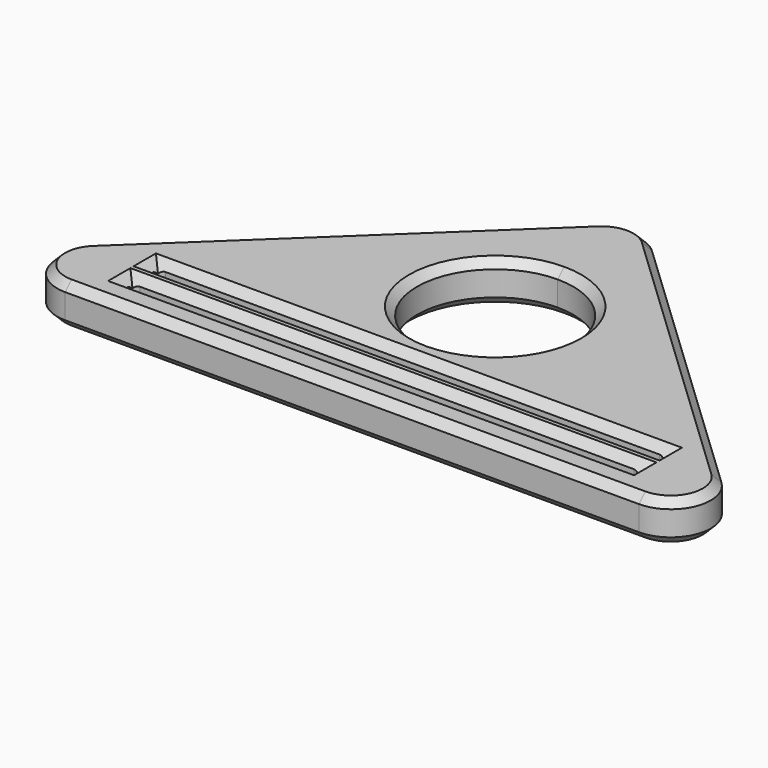
from build123d import *

# Parameters (mm, degrees)
F1_DEPTH      = 5.1
F2_R          = 5
F3_SIZE       = 1
F4_T4_DEPTH   = 8.1
F4_T10_DEPTH  = 8.1
F4_T16_DEPTH  = 8.1
F4_T24_DEPTH  = 8.1
F4_T30_DEPTH  = 8.1
F4_T36_DEPTH  = 8.1
F4_T42_DEPTH  = 8.1
F4_T48_DEPTH  = 8.1
F4_T56_DEPTH  = 8.1
F4_T62_DEPTH  = 8.1
F4_T68_DEPTH  = 8.1
F4_T74_DEPTH  = 8.1
F4_T80_DEPTH  = 8.1
F4_T88_DEPTH  = 8.1
F4_T94_DEPTH  = 8.1
F4_T100_DEPTH = 8.1
F4_T106_DEPTH = 8.1
F4_T112_DEPTH = 8.1
F4_T120_DEPTH = 8.1
F4_T126_DEPTH = 8.1
F4_T132_DEPTH = 8.1
F4_T138_DEPTH = 8.1
F4_T144_DEPTH = 8.1
F4_T152_DEPTH = 8.1
F4_T158_DEPTH = 8.1
F4_T164_DEPTH = 8.1
F4_T170_DEPTH = 8.1
F4_T176_DEPTH = 8.1
F4_T184_DEPTH = 8.1
F4_T190_DEPTH = 8.1
F4_T196_DEPTH = 8.1
F4_T202_DEPTH = 8.1
F4_T208_DEPTH = 8.1
F4_T216_DEPTH = 8.1
F4_T222_DEPTH = 8.1
F4_T228_DEPTH = 8.1
F4_T234_DEPTH = 8.1
F4_T240_DEPTH = 8.1
F4_T248_DEPTH = 8.1
F4_T254_DEPTH = 8.1


# Not quite as in the source:
# - a fillet or chamfer that OpenCascade refuses, or shapes differently, is made with other operations: its cross-section is extruded or revolved along the edge and cut away or added


with BuildPart() as f1:
    # F0 (on Top) → F1 (new body)
    with BuildSketch(Plane.XY):
        with BuildLine():
            Line((0, 2.5), (0, 0))
            Line((0, 0), (32, 0))
            Line((32, 0), (32, -1.5))
            Line((32, -1.5), (0, -1.5))
            Line((0, -1.5), (0, -5.4818979414))
            Line((0, -5.4818979414), (48.5503548798, -5.4818979414))
            Line((48.5503548798, -5.4818979414), (0, 40.5181020586))
            Line((0, 40.5181020586), (0, 26.7715353826))
            ThreePointArc((0, 26.7715353826), (6.9368136311, 23.8982130969), (9.8101359168, 16.9613994658))
            ThreePointArc((9.8101359168, 16.9613994658), (6.9368136311, 10.0245858347), (0, 7.151263549))
            Line((0, 7.151263549), (0, 4))
            Line((0, 4), (32, 4))
            Line((32, 4), (32, 2.5))
            Line((32, 2.5), (0, 2.5))
        make_face()
        with BuildLine():
            Line((-32, -1.5), (-32, 0))
            Line((-32, 0), (0, 0))
            Line((0, 0), (0, 2.5))
            Line((0, 2.5), (-32, 2.5))
            Line((-32, 2.5), (-32, 4))
            Line((-32, 4), (0, 4))
            Line((0, 4), (0, 7.151263549))
            ThreePointArc((0, 7.151263549), (-9.8101359168, 16.9613994658), (0, 26.7715353826))
            Line((0, 26.7715353826), (0, 40.5181020586))
            Line((0, 40.5181020586), (-48.5503548798, -5.4818979414))
            Line((-48.5503548798, -5.4818979414), (0, -5.4818979414))
            Line((0, -5.4818979414), (0, -1.5))
            Line((0, -1.5), (-32, -1.5))
        make_face()
    extrude(amount=F1_DEPTH)

    # F2
    f2_edges = [f1.edges().sort_by_distance(p)[0] for p in [
        (-48.550355, -5.481898, 2.55),
        (48.550355, -5.481898, 2.55),
        (0, 40.518102, 2.55),
    ]]
    fillet(f2_edges, radius=F2_R)

    # F3
    f3_edges = [f1.edges().sort_by_distance(p)[0] for p in [
        (21.440624, 20.203756, 5.1),
        (40.648189, -2.332857, 5.1),
        (0, 38.630252, 5.1),
        (0, -5.481898, 5.1),
        (-21.440624, 20.203756, 5.1),
        (-40.648189, -2.332857, 5.1),
        (32, 3.25, 5.1),
        (0, 2.5, 5.1),
        (-32, 3.25, 5.1),
        (0, 4, 5.1),
        (32, -0.75, 5.1),
        (0, -1.5, 5.1),
        (-32, -0.75, 5.1),
        (0, 0, 5.1),
        (-9.810136, 16.961399, 5.1),
        (21.440624, 20.203756, 0),
        (40.648189, -2.332857, 0),
        (0, 38.630252, 0),
        (0, -5.481898, 0),
        (-21.440624, 20.203756, 0),
        (-40.648189, -2.332857, 0),
        (32, 3.25, 0),
        (0, 2.5, 0),
        (-32, 3.25, 0),
        (0, 4, 0),
        (32, -0.75, 0),
        (0, -1.5, 0),
        (-32, -0.75, 0),
        (0, 0, 0),
        (-9.810136, 16.961399, 0),
    ]]
    chamfer(f3_edges, length=F3_SIZE)

    # F4: fillet of radius 1 on 8 edges, made by hand


with BuildPart() as f4_tool2:
    # F4_s3 → F4_t4 (new body)
    with BuildSketch(Plane.XY.offset(-1.5)):
        with BuildLine():
            ThreePointArc((32, 3.5), (31.7071067812, 2.7928932188), (31, 2.5))
            Line((31, 2.5), (32, 2.5))
            Line((32, 2.5), (32, 3.5))
        make_face()
    extrude(amount=F4_T4_DEPTH)

    split(bisect_by=Plane(origin=(16.5, 0, 16.5), x_dir=(0, 1, 0), z_dir=(-0.7071067812, 0, -0.7071067812)), keep=Keep.TOP)

    split(bisect_by=Plane(origin=(0, 0.75, -0.75), x_dir=(1, 0, 0), z_dir=(0, -0.7071067812, 0.7071067812)), keep=Keep.TOP)


with BuildPart() as f1_1:
    add(f1.part)

    # F4_t1: union F4_tool2
    add(f4_tool2.part)


with BuildPart() as f4_tool8:
    # F4_s9 → F4_t10 (new body)
    with BuildSketch(Plane.XY.offset(-1.5)):
        with BuildLine():
            ThreePointArc((32, 3.5), (31.7071067812, 2.7928932188), (31, 2.5))
            Line((31, 2.5), (32, 2.5))
            Line((32, 2.5), (32, 3.5))
        make_face()
    extrude(amount=F4_T10_DEPTH)

    split(bisect_by=Plane(origin=(16.5, 0, 16.5), x_dir=(0, 1, 0), z_dir=(0.7071067812, 0, 0.7071067812)), keep=Keep.TOP)

    split(bisect_by=Plane(origin=(0, 0.75, -0.75), x_dir=(1, 0, 0), z_dir=(0, 0.7071067812, -0.7071067812)), keep=Keep.TOP)


with BuildPart() as f1_2:
    add(f1_1.part)

    # F4_t7: union F4_tool8
    add(f4_tool8.part)


with BuildPart() as f4_tool14:
    # F4_s15 → F4_t16 (new body)
    with BuildSketch(Plane.XY.offset(-1.5)):
        with BuildLine():
            ThreePointArc((32, 3.5), (31.7071067812, 2.7928932188), (31, 2.5))
            Line((31, 2.5), (32, 2.5))
            Line((32, 2.5), (32, 3.5))
        make_face()
    extrude(amount=F4_T16_DEPTH)

    split(bisect_by=Plane(origin=(16.5, 0, 16.5), x_dir=(0, 1, 0), z_dir=(0.7071067812, 0, 0.7071067812)), keep=Keep.TOP)

    split(bisect_by=Plane(origin=(0, 0.75, -0.75), x_dir=(1, 0, 0), z_dir=(0, -0.7071067812, 0.7071067812)), keep=Keep.TOP)

    split(bisect_by=Plane(origin=(13.95, 0, -13.95), x_dir=(0, 1, 0), z_dir=(0.7071067812, 0, -0.7071067812)), keep=Keep.TOP)

    split(bisect_by=Plane(origin=(0, 3.3, 3.3), x_dir=(1, 0, 0), z_dir=(0, -0.7071067812, -0.7071067812)), keep=Keep.TOP)


with BuildPart() as f1_3:
    add(f1_2.part)

    # F4_t13: union F4_tool14
    add(f4_tool14.part)


with BuildPart() as f4_tool22:
    # F4_s23 → F4_t24 (new body)
    with BuildSketch(Plane.XY.offset(-1.5)):
        with BuildLine():
            ThreePointArc((32, 3.5), (31.7071067812, 2.7928932188), (31, 2.5))
            Line((31, 2.5), (32, 2.5))
            Line((32, 2.5), (32, 3.5))
        make_face()
    extrude(amount=F4_T24_DEPTH)

    split(bisect_by=Plane(origin=(13.95, 0, -13.95), x_dir=(0, 1, 0), z_dir=(-0.7071067812, 0, 0.7071067812)), keep=Keep.TOP)

    split(bisect_by=Plane(origin=(0, 3.3, 3.3), x_dir=(1, 0, 0), z_dir=(0, -0.7071067812, -0.7071067812)), keep=Keep.TOP)


with BuildPart() as f1_4:
    add(f1_3.part)

    # F4_t21: union F4_tool22
    add(f4_tool22.part)


with BuildPart() as f4_tool28:
    # F4_s29 → F4_t30 (new body)
    with BuildSketch(Plane.XY.offset(-1.5)):
        with BuildLine():
            ThreePointArc((32, 3.5), (31.7071067812, 2.7928932188), (31, 2.5))
            Line((31, 2.5), (32, 2.5))
            Line((32, 2.5), (32, 3.5))
        make_face()
    extrude(amount=F4_T30_DEPTH)

    split(bisect_by=Plane(origin=(13.95, 0, -13.95), x_dir=(0, 1, 0), z_dir=(0.7071067812, 0, -0.7071067812)), keep=Keep.TOP)

    split(bisect_by=Plane(origin=(0, 3.3, 3.3), x_dir=(1, 0, 0), z_dir=(0, 0.7071067812, 0.7071067812)), keep=Keep.TOP)


with BuildPart() as f1_5:
    add(f1_4.part)

    # F4_t27: union F4_tool28
    add(f4_tool28.part)


with BuildPart() as f4_tool34:
    # F4_s35 → F4_t36 (new body)
    with BuildSketch(Plane.XY.offset(-1.5)):
        with BuildLine():
            ThreePointArc((32, -1), (31.7071067812, -0.2928932188), (31, 0))
            Line((31, 0), (32, 0))
            Line((32, 0), (32, -1))
        make_face()
    extrude(amount=F4_T36_DEPTH)

    split(bisect_by=Plane(origin=(16.5, 0, 16.5), x_dir=(0, 1, 0), z_dir=(-0.7071067812, 0, -0.7071067812)), keep=Keep.TOP)

    split(bisect_by=Plane(origin=(0, 0.5, 0.5), x_dir=(1, 0, 0), z_dir=(0, 0.7071067812, 0.7071067812)), keep=Keep.TOP)


with BuildPart() as f1_6:
    add(f1_5.part)

    # F4_t33: union F4_tool34
    add(f4_tool34.part)


with BuildPart() as f4_tool40:
    # F4_s41 → F4_t42 (new body)
    with BuildSketch(Plane.XY.offset(-1.5)):
        with BuildLine():
            ThreePointArc((32, -1), (31.7071067812, -0.2928932188), (31, 0))
            Line((31, 0), (32, 0))
            Line((32, 0), (32, -1))
        make_face()
    extrude(amount=F4_T42_DEPTH)

    split(bisect_by=Plane(origin=(16.5, 0, 16.5), x_dir=(0, 1, 0), z_dir=(0.7071067812, 0, 0.7071067812)), keep=Keep.TOP)

    split(bisect_by=Plane(origin=(0, 0.5, 0.5), x_dir=(1, 0, 0), z_dir=(0, -0.7071067812, -0.7071067812)), keep=Keep.TOP)


with BuildPart() as f1_7:
    add(f1_6.part)

    # F4_t39: union F4_tool40
    add(f4_tool40.part)


with BuildPart() as f4_tool46:
    # F4_s47 → F4_t48 (new body)
    with BuildSketch(Plane.XY.offset(-1.5)):
        with BuildLine():
            ThreePointArc((32, -1), (31.7071067812, -0.2928932188), (31, 0))
            Line((31, 0), (32, 0))
            Line((32, 0), (32, -1))
        make_face()
    extrude(amount=F4_T48_DEPTH)

    split(bisect_by=Plane(origin=(16.5, 0, 16.5), x_dir=(0, 1, 0), z_dir=(0.7071067812, 0, 0.7071067812)), keep=Keep.TOP)

    split(bisect_by=Plane(origin=(0, 0.5, 0.5), x_dir=(1, 0, 0), z_dir=(0, 0.7071067812, 0.7071067812)), keep=Keep.TOP)

    split(bisect_by=Plane(origin=(13.95, 0, -13.95), x_dir=(0, 1, 0), z_dir=(0.7071067812, 0, -0.7071067812)), keep=Keep.TOP)

    split(bisect_by=Plane(origin=(0, -2.05, 2.05), x_dir=(1, 0, 0), z_dir=(0, 0.7071067812, -0.7071067812)), keep=Keep.TOP)


with BuildPart() as f1_8:
    add(f1_7.part)

    # F4_t45: union F4_tool46
    add(f4_tool46.part)


with BuildPart() as f4_tool54:
    # F4_s55 → F4_t56 (new body)
    with BuildSketch(Plane.XY.offset(-1.5)):
        with BuildLine():
            ThreePointArc((32, -1), (31.7071067812, -0.2928932188), (31, 0))
            Line((31, 0), (32, 0))
            Line((32, 0), (32, -1))
        make_face()
    extrude(amount=F4_T56_DEPTH)

    split(bisect_by=Plane(origin=(13.95, 0, -13.95), x_dir=(0, 1, 0), z_dir=(-0.7071067812, 0, 0.7071067812)), keep=Keep.TOP)

    split(bisect_by=Plane(origin=(0, -2.05, 2.05), x_dir=(1, 0, 0), z_dir=(0, 0.7071067812, -0.7071067812)), keep=Keep.TOP)


with BuildPart() as f1_9:
    add(f1_8.part)

    # F4_t53: union F4_tool54
    add(f4_tool54.part)


with BuildPart() as f4_tool60:
    # F4_s61 → F4_t62 (new body)
    with BuildSketch(Plane.XY.offset(-1.5)):
        with BuildLine():
            ThreePointArc((32, -1), (31.7071067812, -0.2928932188), (31, 0))
            Line((31, 0), (32, 0))
            Line((32, 0), (32, -1))
        make_face()
    extrude(amount=F4_T62_DEPTH)

    split(bisect_by=Plane(origin=(13.95, 0, -13.95), x_dir=(0, 1, 0), z_dir=(0.7071067812, 0, -0.7071067812)), keep=Keep.TOP)

    split(bisect_by=Plane(origin=(0, -2.05, 2.05), x_dir=(1, 0, 0), z_dir=(0, -0.7071067812, 0.7071067812)), keep=Keep.TOP)


with BuildPart() as f1_10:
    add(f1_9.part)

    # F4_t59: union F4_tool60
    add(f4_tool60.part)


with BuildPart() as f4_tool66:
    # F4_s67 → F4_t68 (new body)
    with BuildSketch(Plane.XY.offset(-1.5)):
        with BuildLine():
            ThreePointArc((32, -0.5), (31.7071067812, -1.2071067812), (31, -1.5))
            Line((31, -1.5), (32, -1.5))
            Line((32, -1.5), (32, -0.5))
        make_face()
    extrude(amount=F4_T68_DEPTH)

    split(bisect_by=Plane(origin=(16.5, 0, 16.5), x_dir=(0, 1, 0), z_dir=(-0.7071067812, 0, -0.7071067812)), keep=Keep.TOP)

    split(bisect_by=Plane(origin=(0, -1.25, 1.25), x_dir=(1, 0, 0), z_dir=(0, -0.7071067812, 0.7071067812)), keep=Keep.TOP)


with BuildPart() as f1_11:
    add(f1_10.part)

    # F4_t65: union F4_tool66
    add(f4_tool66.part)


with BuildPart() as f4_tool72:
    # F4_s73 → F4_t74 (new body)
    with BuildSketch(Plane.XY.offset(-1.5)):
        with BuildLine():
            ThreePointArc((32, -0.5), (31.7071067812, -1.2071067812), (31, -1.5))
            Line((31, -1.5), (32, -1.5))
            Line((32, -1.5), (32, -0.5))
        make_face()
    extrude(amount=F4_T74_DEPTH)

    split(bisect_by=Plane(origin=(16.5, 0, 16.5), x_dir=(0, 1, 0), z_dir=(0.7071067812, 0, 0.7071067812)), keep=Keep.TOP)

    split(bisect_by=Plane(origin=(0, -1.25, 1.25), x_dir=(1, 0, 0), z_dir=(0, 0.7071067812, -0.7071067812)), keep=Keep.TOP)


with BuildPart() as f1_12:
    add(f1_11.part)

    # F4_t71: union F4_tool72
    add(f4_tool72.part)


with BuildPart() as f4_tool78:
    # F4_s79 → F4_t80 (new body)
    with BuildSketch(Plane.XY.offset(-1.5)):
        with BuildLine():
            ThreePointArc((32, -0.5), (31.7071067812, -1.2071067812), (31, -1.5))
            Line((31, -1.5), (32, -1.5))
            Line((32, -1.5), (32, -0.5))
        make_face()
    extrude(amount=F4_T80_DEPTH)

    split(bisect_by=Plane(origin=(16.5, 0, 16.5), x_dir=(0, 1, 0), z_dir=(0.7071067812, 0, 0.7071067812)), keep=Keep.TOP)

    split(bisect_by=Plane(origin=(0, -1.25, 1.25), x_dir=(1, 0, 0), z_dir=(0, -0.7071067812, 0.7071067812)), keep=Keep.TOP)

    split(bisect_by=Plane(origin=(13.95, 0, -13.95), x_dir=(0, 1, 0), z_dir=(0.7071067812, 0, -0.7071067812)), keep=Keep.TOP)

    split(bisect_by=Plane(origin=(0, 1.3, 1.3), x_dir=(1, 0, 0), z_dir=(0, -0.7071067812, -0.7071067812)), keep=Keep.TOP)


with BuildPart() as f1_13:
    add(f1_12.part)

    # F4_t77: union F4_tool78
    add(f4_tool78.part)


with BuildPart() as f4_tool86:
    # F4_s87 → F4_t88 (new body)
    with BuildSketch(Plane.XY.offset(-1.5)):
        with BuildLine():
            ThreePointArc((32, -0.5), (31.7071067812, -1.2071067812), (31, -1.5))
            Line((31, -1.5), (32, -1.5))
            Line((32, -1.5), (32, -0.5))
        make_face()
    extrude(amount=F4_T88_DEPTH)

    split(bisect_by=Plane(origin=(13.95, 0, -13.95), x_dir=(0, 1, 0), z_dir=(-0.7071067812, 0, 0.7071067812)), keep=Keep.TOP)

    split(bisect_by=Plane(origin=(0, 1.3, 1.3), x_dir=(1, 0, 0), z_dir=(0, -0.7071067812, -0.7071067812)), keep=Keep.TOP)


with BuildPart() as f1_14:
    add(f1_13.part)

    # F4_t85: union F4_tool86
    add(f4_tool86.part)


with BuildPart() as f4_tool92:
    # F4_s93 → F4_t94 (new body)
    with BuildSketch(Plane.XY.offset(-1.5)):
        with BuildLine():
            ThreePointArc((32, -0.5), (31.7071067812, -1.2071067812), (31, -1.5))
            Line((31, -1.5), (32, -1.5))
            Line((32, -1.5), (32, -0.5))
        make_face()
    extrude(amount=F4_T94_DEPTH)

    split(bisect_by=Plane(origin=(13.95, 0, -13.95), x_dir=(0, 1, 0), z_dir=(0.7071067812, 0, -0.7071067812)), keep=Keep.TOP)

    split(bisect_by=Plane(origin=(0, 1.3, 1.3), x_dir=(1, 0, 0), z_dir=(0, 0.7071067812, 0.7071067812)), keep=Keep.TOP)


with BuildPart() as f1_15:
    add(f1_14.part)

    # F4_t91: union F4_tool92
    add(f4_tool92.part)


with BuildPart() as f4_tool98:
    # F4_s99 → F4_t100 (new body)
    with BuildSketch(Plane.XY.offset(-1.5)):
        with BuildLine():
            ThreePointArc((32, 3), (31.7071067812, 3.7071067812), (31, 4))
            Line((31, 4), (32, 4))
            Line((32, 4), (32, 3))
        make_face()
    extrude(amount=F4_T100_DEPTH)

    split(bisect_by=Plane(origin=(16.5, 0, 16.5), x_dir=(0, 1, 0), z_dir=(-0.7071067812, 0, -0.7071067812)), keep=Keep.TOP)

    split(bisect_by=Plane(origin=(0, 2.5, 2.5), x_dir=(1, 0, 0), z_dir=(0, 0.7071067812, 0.7071067812)), keep=Keep.TOP)


with BuildPart() as f1_16:
    add(f1_15.part)

    # F4_t97: union F4_tool98
    add(f4_tool98.part)


with BuildPart() as f4_tool104:
    # F4_s105 → F4_t106 (new body)
    with BuildSketch(Plane.XY.offset(-1.5)):
        with BuildLine():
            ThreePointArc((32, 3), (31.7071067812, 3.7071067812), (31, 4))
            Line((31, 4), (32, 4))
            Line((32, 4), (32, 3))
        make_face()
    extrude(amount=F4_T106_DEPTH)

    split(bisect_by=Plane(origin=(16.5, 0, 16.5), x_dir=(0, 1, 0), z_dir=(0.7071067812, 0, 0.7071067812)), keep=Keep.TOP)

    split(bisect_by=Plane(origin=(0, 2.5, 2.5), x_dir=(1, 0, 0), z_dir=(0, -0.7071067812, -0.7071067812)), keep=Keep.TOP)


with BuildPart() as f1_17:
    add(f1_16.part)

    # F4_t103: union F4_tool104
    add(f4_tool104.part)


with BuildPart() as f4_tool110:
    # F4_s111 → F4_t112 (new body)
    with BuildSketch(Plane.XY.offset(-1.5)):
        with BuildLine():
            ThreePointArc((32, 3), (31.7071067812, 3.7071067812), (31, 4))
            Line((31, 4), (32, 4))
            Line((32, 4), (32, 3))
        make_face()
    extrude(amount=F4_T112_DEPTH)

    split(bisect_by=Plane(origin=(16.5, 0, 16.5), x_dir=(0, 1, 0), z_dir=(0.7071067812, 0, 0.7071067812)), keep=Keep.TOP)

    split(bisect_by=Plane(origin=(0, 2.5, 2.5), x_dir=(1, 0, 0), z_dir=(0, 0.7071067812, 0.7071067812)), keep=Keep.TOP)

    split(bisect_by=Plane(origin=(13.95, 0, -13.95), x_dir=(0, 1, 0), z_dir=(0.7071067812, 0, -0.7071067812)), keep=Keep.TOP)

    split(bisect_by=Plane(origin=(0, -0.05, 0.05), x_dir=(1, 0, 0), z_dir=(0, 0.7071067812, -0.7071067812)), keep=Keep.TOP)


with BuildPart() as f1_18:
    add(f1_17.part)

    # F4_t109: union F4_tool110
    add(f4_tool110.part)


with BuildPart() as f4_tool118:
    # F4_s119 → F4_t120 (new body)
    with BuildSketch(Plane.XY.offset(-1.5)):
        with BuildLine():
            ThreePointArc((32, 3), (31.7071067812, 3.7071067812), (31, 4))
            Line((31, 4), (32, 4))
            Line((32, 4), (32, 3))
        make_face()
    extrude(amount=F4_T120_DEPTH)

    split(bisect_by=Plane(origin=(13.95, 0, -13.95), x_dir=(0, 1, 0), z_dir=(-0.7071067812, 0, 0.7071067812)), keep=Keep.TOP)

    split(bisect_by=Plane(origin=(0, -0.05, 0.05), x_dir=(1, 0, 0), z_dir=(0, 0.7071067812, -0.7071067812)), keep=Keep.TOP)


with BuildPart() as f1_19:
    add(f1_18.part)

    # F4_t117: union F4_tool118
    add(f4_tool118.part)


with BuildPart() as f4_tool124:
    # F4_s125 → F4_t126 (new body)
    with BuildSketch(Plane.XY.offset(-1.5)):
        with BuildLine():
            ThreePointArc((32, 3), (31.7071067812, 3.7071067812), (31, 4))
            Line((31, 4), (32, 4))
            Line((32, 4), (32, 3))
        make_face()
    extrude(amount=F4_T126_DEPTH)

    split(bisect_by=Plane(origin=(13.95, 0, -13.95), x_dir=(0, 1, 0), z_dir=(0.7071067812, 0, -0.7071067812)), keep=Keep.TOP)

    split(bisect_by=Plane(origin=(0, -0.05, 0.05), x_dir=(1, 0, 0), z_dir=(0, -0.7071067812, 0.7071067812)), keep=Keep.TOP)


with BuildPart() as f1_20:
    add(f1_19.part)

    # F4_t123: union F4_tool124
    add(f4_tool124.part)


with BuildPart() as f4_tool130:
    # F4_s131 → F4_t132 (new body)
    with BuildSketch(Plane.XY.offset(-1.5)):
        with BuildLine():
            ThreePointArc((-31, -1.5), (-31.7071067812, -1.2071067812), (-32, -0.5))
            Line((-32, -0.5), (-32, -1.5))
            Line((-32, -1.5), (-31, -1.5))
        make_face()
    extrude(amount=F4_T132_DEPTH)

    split(bisect_by=Plane(origin=(0, -1.25, 1.25), x_dir=(1, 0, 0), z_dir=(0, 0.7071067812, -0.7071067812)), keep=Keep.TOP)

    split(bisect_by=Plane(origin=(-16.5, 0, 16.5), x_dir=(0, 1, 0), z_dir=(-0.7071067812, 0, 0.7071067812)), keep=Keep.TOP)


with BuildPart() as f1_21:
    add(f1_20.part)

    # F4_t129: union F4_tool130
    add(f4_tool130.part)


with BuildPart() as f4_tool136:
    # F4_s137 → F4_t138 (new body)
    with BuildSketch(Plane.XY.offset(-1.5)):
        with BuildLine():
            ThreePointArc((-31, -1.5), (-31.7071067812, -1.2071067812), (-32, -0.5))
            Line((-32, -0.5), (-32, -1.5))
            Line((-32, -1.5), (-31, -1.5))
        make_face()
    extrude(amount=F4_T138_DEPTH)

    split(bisect_by=Plane(origin=(0, -1.25, 1.25), x_dir=(1, 0, 0), z_dir=(0, -0.7071067812, 0.7071067812)), keep=Keep.TOP)

    split(bisect_by=Plane(origin=(-16.5, 0, 16.5), x_dir=(0, 1, 0), z_dir=(0.7071067812, 0, -0.7071067812)), keep=Keep.TOP)


with BuildPart() as f1_22:
    add(f1_21.part)

    # F4_t135: union F4_tool136
    add(f4_tool136.part)


with BuildPart() as f4_tool142:
    # F4_s143 → F4_t144 (new body)
    with BuildSketch(Plane.XY.offset(-1.5)):
        with BuildLine():
            ThreePointArc((-31, -1.5), (-31.7071067812, -1.2071067812), (-32, -0.5))
            Line((-32, -0.5), (-32, -1.5))
            Line((-32, -1.5), (-31, -1.5))
        make_face()
    extrude(amount=F4_T144_DEPTH)

    split(bisect_by=Plane(origin=(0, -1.25, 1.25), x_dir=(1, 0, 0), z_dir=(0, -0.7071067812, 0.7071067812)), keep=Keep.TOP)

    split(bisect_by=Plane(origin=(-16.5, 0, 16.5), x_dir=(0, 1, 0), z_dir=(-0.7071067812, 0, 0.7071067812)), keep=Keep.TOP)

    split(bisect_by=Plane(origin=(0, 1.3, 1.3), x_dir=(1, 0, 0), z_dir=(0, -0.7071067812, -0.7071067812)), keep=Keep.TOP)

    split(bisect_by=Plane(origin=(-13.95, 0, -13.95), x_dir=(0, 1, 0), z_dir=(-0.7071067812, 0, -0.7071067812)), keep=Keep.TOP)


with BuildPart() as f1_23:
    add(f1_22.part)

    # F4_t141: union F4_tool142
    add(f4_tool142.part)


with BuildPart() as f4_tool150:
    # F4_s151 → F4_t152 (new body)
    with BuildSketch(Plane.XY.offset(-1.5)):
        with BuildLine():
            ThreePointArc((-31, -1.5), (-31.7071067812, -1.2071067812), (-32, -0.5))
            Line((-32, -0.5), (-32, -1.5))
            Line((-32, -1.5), (-31, -1.5))
        make_face()
    extrude(amount=F4_T152_DEPTH)

    split(bisect_by=Plane(origin=(0, 1.3, 1.3), x_dir=(1, 0, 0), z_dir=(0, 0.7071067812, 0.7071067812)), keep=Keep.TOP)

    split(bisect_by=Plane(origin=(-13.95, 0, -13.95), x_dir=(0, 1, 0), z_dir=(-0.7071067812, 0, -0.7071067812)), keep=Keep.TOP)


with BuildPart() as f1_24:
    add(f1_23.part)

    # F4_t149: union F4_tool150
    add(f4_tool150.part)


with BuildPart() as f4_tool156:
    # F4_s157 → F4_t158 (new body)
    with BuildSketch(Plane.XY.offset(-1.5)):
        with BuildLine():
            ThreePointArc((-31, -1.5), (-31.7071067812, -1.2071067812), (-32, -0.5))
            Line((-32, -0.5), (-32, -1.5))
            Line((-32, -1.5), (-31, -1.5))
        make_face()
    extrude(amount=F4_T158_DEPTH)

    split(bisect_by=Plane(origin=(0, 1.3, 1.3), x_dir=(1, 0, 0), z_dir=(0, -0.7071067812, -0.7071067812)), keep=Keep.TOP)

    split(bisect_by=Plane(origin=(-13.95, 0, -13.95), x_dir=(0, 1, 0), z_dir=(0.7071067812, 0, 0.7071067812)), keep=Keep.TOP)


with BuildPart() as f1_25:
    add(f1_24.part)

    # F4_t155: union F4_tool156
    add(f4_tool156.part)


with BuildPart() as f4_tool162:
    # F4_s163 → F4_t164 (new body)
    with BuildSketch(Plane.XY.offset(-1.5)):
        with BuildLine():
            ThreePointArc((-31, 2.5), (-31.7071067812, 2.7928932188), (-32, 3.5))
            Line((-32, 3.5), (-32, 2.5))
            Line((-32, 2.5), (-31, 2.5))
        make_face()
    extrude(amount=F4_T164_DEPTH)

    split(bisect_by=Plane(origin=(0, 0.75, -0.75), x_dir=(1, 0, 0), z_dir=(0, 0.7071067812, -0.7071067812)), keep=Keep.TOP)

    split(bisect_by=Plane(origin=(-16.5, 0, 16.5), x_dir=(0, 1, 0), z_dir=(-0.7071067812, 0, 0.7071067812)), keep=Keep.TOP)


with BuildPart() as f1_26:
    add(f1_25.part)

    # F4_t161: union F4_tool162
    add(f4_tool162.part)


with BuildPart() as f4_tool168:
    # F4_s169 → F4_t170 (new body)
    with BuildSketch(Plane.XY.offset(-1.5)):
        with BuildLine():
            ThreePointArc((-31, 2.5), (-31.7071067812, 2.7928932188), (-32, 3.5))
            Line((-32, 3.5), (-32, 2.5))
            Line((-32, 2.5), (-31, 2.5))
        make_face()
    extrude(amount=F4_T170_DEPTH)

    split(bisect_by=Plane(origin=(0, 0.75, -0.75), x_dir=(1, 0, 0), z_dir=(0, -0.7071067812, 0.7071067812)), keep=Keep.TOP)

    split(bisect_by=Plane(origin=(-16.5, 0, 16.5), x_dir=(0, 1, 0), z_dir=(0.7071067812, 0, -0.7071067812)), keep=Keep.TOP)


with BuildPart() as f1_27:
    add(f1_26.part)

    # F4_t167: union F4_tool168
    add(f4_tool168.part)


with BuildPart() as f4_tool174:
    # F4_s175 → F4_t176 (new body)
    with BuildSketch(Plane.XY.offset(-1.5)):
        with BuildLine():
            ThreePointArc((-31, 2.5), (-31.7071067812, 2.7928932188), (-32, 3.5))
            Line((-32, 3.5), (-32, 2.5))
            Line((-32, 2.5), (-31, 2.5))
        make_face()
    extrude(amount=F4_T176_DEPTH)

    split(bisect_by=Plane(origin=(0, 0.75, -0.75), x_dir=(1, 0, 0), z_dir=(0, -0.7071067812, 0.7071067812)), keep=Keep.TOP)

    split(bisect_by=Plane(origin=(-16.5, 0, 16.5), x_dir=(0, 1, 0), z_dir=(-0.7071067812, 0, 0.7071067812)), keep=Keep.TOP)

    split(bisect_by=Plane(origin=(0, 3.3, 3.3), x_dir=(1, 0, 0), z_dir=(0, -0.7071067812, -0.7071067812)), keep=Keep.TOP)

    split(bisect_by=Plane(origin=(-13.95, 0, -13.95), x_dir=(0, 1, 0), z_dir=(-0.7071067812, 0, -0.7071067812)), keep=Keep.TOP)


with BuildPart() as f1_28:
    add(f1_27.part)

    # F4_t173: union F4_tool174
    add(f4_tool174.part)


with BuildPart() as f4_tool182:
    # F4_s183 → F4_t184 (new body)
    with BuildSketch(Plane.XY.offset(-1.5)):
        with BuildLine():
            ThreePointArc((-31, 2.5), (-31.7071067812, 2.7928932188), (-32, 3.5))
            Line((-32, 3.5), (-32, 2.5))
            Line((-32, 2.5), (-31, 2.5))
        make_face()
    extrude(amount=F4_T184_DEPTH)

    split(bisect_by=Plane(origin=(0, 3.3, 3.3), x_dir=(1, 0, 0), z_dir=(0, 0.7071067812, 0.7071067812)), keep=Keep.TOP)

    split(bisect_by=Plane(origin=(-13.95, 0, -13.95), x_dir=(0, 1, 0), z_dir=(-0.7071067812, 0, -0.7071067812)), keep=Keep.TOP)


with BuildPart() as f1_29:
    add(f1_28.part)

    # F4_t181: union F4_tool182
    add(f4_tool182.part)


with BuildPart() as f4_tool188:
    # F4_s189 → F4_t190 (new body)
    with BuildSketch(Plane.XY.offset(-1.5)):
        with BuildLine():
            ThreePointArc((-31, 2.5), (-31.7071067812, 2.7928932188), (-32, 3.5))
            Line((-32, 3.5), (-32, 2.5))
            Line((-32, 2.5), (-31, 2.5))
        make_face()
    extrude(amount=F4_T190_DEPTH)

    split(bisect_by=Plane(origin=(0, 3.3, 3.3), x_dir=(1, 0, 0), z_dir=(0, -0.7071067812, -0.7071067812)), keep=Keep.TOP)

    split(bisect_by=Plane(origin=(-13.95, 0, -13.95), x_dir=(0, 1, 0), z_dir=(0.7071067812, 0, 0.7071067812)), keep=Keep.TOP)


with BuildPart() as f1_30:
    add(f1_29.part)

    # F4_t187: union F4_tool188
    add(f4_tool188.part)


with BuildPart() as f4_tool194:
    # F4_s195 → F4_t196 (new body)
    with BuildSketch(Plane.XY.offset(-1.5)):
        with BuildLine():
            ThreePointArc((-31, 4), (-31.7071067812, 3.7071067812), (-32, 3))
            Line((-32, 3), (-32, 4))
            Line((-32, 4), (-31, 4))
        make_face()
    extrude(amount=F4_T196_DEPTH)

    split(bisect_by=Plane(origin=(0, 2.5, 2.5), x_dir=(1, 0, 0), z_dir=(0, -0.7071067812, -0.7071067812)), keep=Keep.TOP)

    split(bisect_by=Plane(origin=(-16.5, 0, 16.5), x_dir=(0, 1, 0), z_dir=(-0.7071067812, 0, 0.7071067812)), keep=Keep.TOP)


with BuildPart() as f1_31:
    add(f1_30.part)

    # F4_t193: union F4_tool194
    add(f4_tool194.part)


with BuildPart() as f4_tool200:
    # F4_s201 → F4_t202 (new body)
    with BuildSketch(Plane.XY.offset(-1.5)):
        with BuildLine():
            ThreePointArc((-31, 4), (-31.7071067812, 3.7071067812), (-32, 3))
            Line((-32, 3), (-32, 4))
            Line((-32, 4), (-31, 4))
        make_face()
    extrude(amount=F4_T202_DEPTH)

    split(bisect_by=Plane(origin=(0, 2.5, 2.5), x_dir=(1, 0, 0), z_dir=(0, 0.7071067812, 0.7071067812)), keep=Keep.TOP)

    split(bisect_by=Plane(origin=(-16.5, 0, 16.5), x_dir=(0, 1, 0), z_dir=(0.7071067812, 0, -0.7071067812)), keep=Keep.TOP)


with BuildPart() as f1_32:
    add(f1_31.part)

    # F4_t199: union F4_tool200
    add(f4_tool200.part)


with BuildPart() as f4_tool206:
    # F4_s207 → F4_t208 (new body)
    with BuildSketch(Plane.XY.offset(-1.5)):
        with BuildLine():
            ThreePointArc((-31, 4), (-31.7071067812, 3.7071067812), (-32, 3))
            Line((-32, 3), (-32, 4))
            Line((-32, 4), (-31, 4))
        make_face()
    extrude(amount=F4_T208_DEPTH)

    split(bisect_by=Plane(origin=(0, 2.5, 2.5), x_dir=(1, 0, 0), z_dir=(0, 0.7071067812, 0.7071067812)), keep=Keep.TOP)

    split(bisect_by=Plane(origin=(-16.5, 0, 16.5), x_dir=(0, 1, 0), z_dir=(-0.7071067812, 0, 0.7071067812)), keep=Keep.TOP)

    split(bisect_by=Plane(origin=(0, -0.05, 0.05), x_dir=(1, 0, 0), z_dir=(0, 0.7071067812, -0.7071067812)), keep=Keep.TOP)

    split(bisect_by=Plane(origin=(-13.95, 0, -13.95), x_dir=(0, 1, 0), z_dir=(-0.7071067812, 0, -0.7071067812)), keep=Keep.TOP)


with BuildPart() as f1_33:
    add(f1_32.part)

    # F4_t205: union F4_tool206
    add(f4_tool206.part)


with BuildPart() as f4_tool214:
    # F4_s215 → F4_t216 (new body)
    with BuildSketch(Plane.XY.offset(-1.5)):
        with BuildLine():
            ThreePointArc((-31, 4), (-31.7071067812, 3.7071067812), (-32, 3))
            Line((-32, 3), (-32, 4))
            Line((-32, 4), (-31, 4))
        make_face()
    extrude(amount=F4_T216_DEPTH)

    split(bisect_by=Plane(origin=(0, -0.05, 0.05), x_dir=(1, 0, 0), z_dir=(0, -0.7071067812, 0.7071067812)), keep=Keep.TOP)

    split(bisect_by=Plane(origin=(-13.95, 0, -13.95), x_dir=(0, 1, 0), z_dir=(-0.7071067812, 0, -0.7071067812)), keep=Keep.TOP)


with BuildPart() as f1_34:
    add(f1_33.part)

    # F4_t213: union F4_tool214
    add(f4_tool214.part)


with BuildPart() as f4_tool220:
    # F4_s221 → F4_t222 (new body)
    with BuildSketch(Plane.XY.offset(-1.5)):
        with BuildLine():
            ThreePointArc((-31, 4), (-31.7071067812, 3.7071067812), (-32, 3))
            Line((-32, 3), (-32, 4))
            Line((-32, 4), (-31, 4))
        make_face()
    extrude(amount=F4_T222_DEPTH)

    split(bisect_by=Plane(origin=(0, -0.05, 0.05), x_dir=(1, 0, 0), z_dir=(0, 0.7071067812, -0.7071067812)), keep=Keep.TOP)

    split(bisect_by=Plane(origin=(-13.95, 0, -13.95), x_dir=(0, 1, 0), z_dir=(0.7071067812, 0, 0.7071067812)), keep=Keep.TOP)


with BuildPart() as f1_35:
    add(f1_34.part)

    # F4_t219: union F4_tool220
    add(f4_tool220.part)


with BuildPart() as f4_tool226:
    # F4_s227 → F4_t228 (new body)
    with BuildSketch(Plane.XY.offset(-1.5)):
        with BuildLine():
            ThreePointArc((-31, 0), (-31.7071067812, -0.2928932188), (-32, -1))
            Line((-32, -1), (-32, 0))
            Line((-32, 0), (-31, 0))
        make_face()
    extrude(amount=F4_T228_DEPTH)

    split(bisect_by=Plane(origin=(0, 0.5, 0.5), x_dir=(1, 0, 0), z_dir=(0, -0.7071067812, -0.7071067812)), keep=Keep.TOP)

    split(bisect_by=Plane(origin=(-16.5, 0, 16.5), x_dir=(0, 1, 0), z_dir=(-0.7071067812, 0, 0.7071067812)), keep=Keep.TOP)


with BuildPart() as f1_36:
    add(f1_35.part)

    # F4_t225: union F4_tool226
    add(f4_tool226.part)


with BuildPart() as f4_tool232:
    # F4_s233 → F4_t234 (new body)
    with BuildSketch(Plane.XY.offset(-1.5)):
        with BuildLine():
            ThreePointArc((-31, 0), (-31.7071067812, -0.2928932188), (-32, -1))
            Line((-32, -1), (-32, 0))
            Line((-32, 0), (-31, 0))
        make_face()
    extrude(amount=F4_T234_DEPTH)

    split(bisect_by=Plane(origin=(0, 0.5, 0.5), x_dir=(1, 0, 0), z_dir=(0, 0.7071067812, 0.7071067812)), keep=Keep.TOP)

    split(bisect_by=Plane(origin=(-16.5, 0, 16.5), x_dir=(0, 1, 0), z_dir=(0.7071067812, 0, -0.7071067812)), keep=Keep.TOP)


with BuildPart() as f1_37:
    add(f1_36.part)

    # F4_t231: union F4_tool232
    add(f4_tool232.part)


with BuildPart() as f4_tool238:
    # F4_s239 → F4_t240 (new body)
    with BuildSketch(Plane.XY.offset(-1.5)):
        with BuildLine():
            ThreePointArc((-31, 0), (-31.7071067812, -0.2928932188), (-32, -1))
            Line((-32, -1), (-32, 0))
            Line((-32, 0), (-31, 0))
        make_face()
    extrude(amount=F4_T240_DEPTH)

    split(bisect_by=Plane(origin=(0, 0.5, 0.5), x_dir=(1, 0, 0), z_dir=(0, 0.7071067812, 0.7071067812)), keep=Keep.TOP)

    split(bisect_by=Plane(origin=(-16.5, 0, 16.5), x_dir=(0, 1, 0), z_dir=(-0.7071067812, 0, 0.7071067812)), keep=Keep.TOP)

    split(bisect_by=Plane(origin=(0, -2.05, 2.05), x_dir=(1, 0, 0), z_dir=(0, 0.7071067812, -0.7071067812)), keep=Keep.TOP)

    split(bisect_by=Plane(origin=(-13.95, 0, -13.95), x_dir=(0, 1, 0), z_dir=(-0.7071067812, 0, -0.7071067812)), keep=Keep.TOP)


with BuildPart() as f1_38:
    add(f1_37.part)

    # F4_t237: union F4_tool238
    add(f4_tool238.part)


with BuildPart() as f4_tool246:
    # F4_s247 → F4_t248 (new body)
    with BuildSketch(Plane.XY.offset(-1.5)):
        with BuildLine():
            ThreePointArc((-31, 0), (-31.7071067812, -0.2928932188), (-32, -1))
            Line((-32, -1), (-32, 0))
            Line((-32, 0), (-31, 0))
        make_face()
    extrude(amount=F4_T248_DEPTH)

    split(bisect_by=Plane(origin=(0, -2.05, 2.05), x_dir=(1, 0, 0), z_dir=(0, -0.7071067812, 0.7071067812)), keep=Keep.TOP)

    split(bisect_by=Plane(origin=(-13.95, 0, -13.95), x_dir=(0, 1, 0), z_dir=(-0.7071067812, 0, -0.7071067812)), keep=Keep.TOP)


with BuildPart() as f1_39:
    add(f1_38.part)

    # F4_t245: union F4_tool246
    add(f4_tool246.part)


with BuildPart() as f4_tool252:
    # F4_s253 → F4_t254 (new body)
    with BuildSketch(Plane.XY.offset(-1.5)):
        with BuildLine():
            ThreePointArc((-31, 0), (-31.7071067812, -0.2928932188), (-32, -1))
            Line((-32, -1), (-32, 0))
            Line((-32, 0), (-31, 0))
        make_face()
    extrude(amount=F4_T254_DEPTH)

    split(bisect_by=Plane(origin=(0, -2.05, 2.05), x_dir=(1, 0, 0), z_dir=(0, 0.7071067812, -0.7071067812)), keep=Keep.TOP)

    split(bisect_by=Plane(origin=(-13.95, 0, -13.95), x_dir=(0, 1, 0), z_dir=(0.7071067812, 0, 0.7071067812)), keep=Keep.TOP)


with BuildPart() as f1_40:
    add(f1_39.part)

    # F4_t251: union F4_tool252
    add(f4_tool252.part)


solid = f1_40.part
